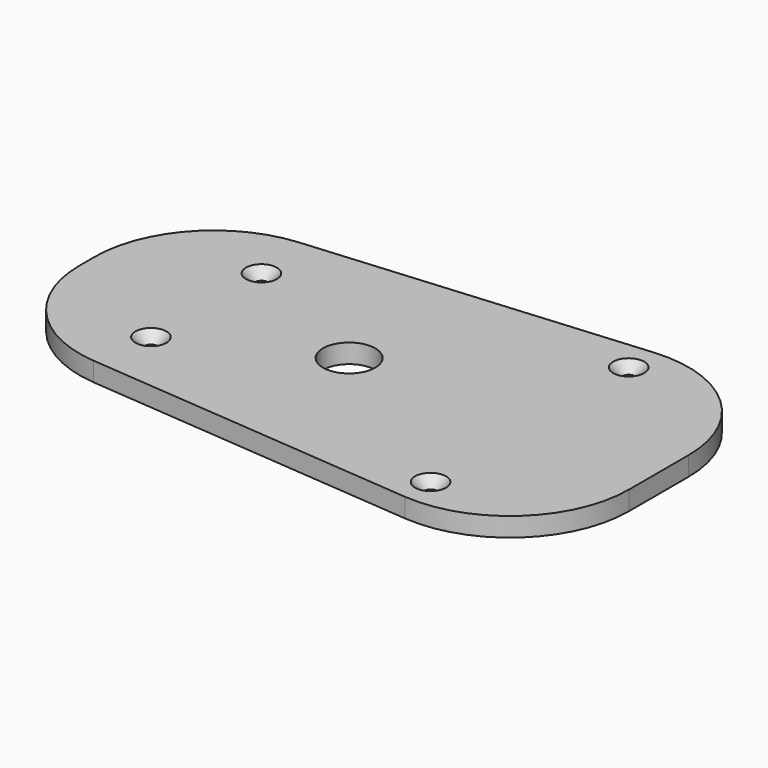
from build123d import *

# Parameters (mm, degrees)
F0_R     = 1.25
F0_R_2   = 5.5
F1_DEPTH = 4
F3_DEPTH = 2
F4_SIZE  = 2


# Not quite as in the source:
# - a feature names something its author has since deleted; it is built from what else it names


with BuildPart() as f1:
    # F0 (on Top) → F1 (new body)
    with BuildSketch(Plane.XY):
        with BuildLine():
            ThreePointArc((-36.0336562554, 5.4360876058), (-41.0336562554, 10.4360876058), (-46.0336562554, 5.4360876058))
            ThreePointArc((-46.0336562554, 5.4360876058), (-48.7113140605, 0.9910484741), (-53.6336562554, -0.6517453414))
            Line((-53.6336562554, -0.6517453414), (-57.6336562554, -0.6517453414))
            Line((-57.6336562554, -0.6517453414), (-59.4336562554, -0.6517453414))
            Line((-59.4336562554, -0.6517453414), (-59.4336562554, -1.3484233022))
            ThreePointArc((-59.4336562554, -1.3484233022), (-52.8307134237, -18.2761605269), (-36.5097932518, -26.2620672584))
            Line((-36.5097932518, -26.2620672584), (33.4902067482, -32.0954005917))
            ThreePointArc((33.4902067482, -32.0954005917), (52.4940809692, -25.5788138039), (60.5663437446, -7.1817566356))
            Line((60.5663437446, -7.1817566356), (60.5663437446, 8.4782659528))
            ThreePointArc((60.5663437446, 8.4782659528), (52.4940809692, 26.8753231211), (33.4902067482, 33.3919099089))
            Line((33.4902067482, 33.3919099089), (-36.5097932518, 27.5585765756))
            ThreePointArc((-36.5097932518, 27.5585765756), (-52.8307134237, 19.5726698441), (-59.4336562554, 2.6449326195))
            Line((-59.4336562554, 2.6449326195), (-59.4336562554, 1.9482546586))
            Line((-59.4336562554, 1.9482546586), (-57.6336562554, 1.9482546586))
            Line((-57.6336562554, 1.9482546586), (-53.6336562554, 1.9482546586))
            ThreePointArc((-53.6336562554, 1.9482546586), (-50.3543429782, 2.8450290737), (-48.4065189788, 5.6314392355))
            ThreePointArc((-48.4065189788, 5.6314392355), (-40.8279863477, 12.5929298404), (-33.4336562554, 5.4360876058))
            ThreePointArc((-33.4336562554, 5.4360876058), (-31.5267024615, 2.8420068396), (-28.4336562554, 1.9482546586))
            Line((-28.4336562554, 1.9482546586), (-15.4336562554, 1.9482546586))
            Line((-15.4336562554, 1.9482546586), (-15.4336562554, 15.2482546586))
            Line((-15.4336562554, 15.2482546586), (-4.9336562554, 15.2482546586))
            Line((-4.9336562554, 15.2482546586), (-4.9336562554, 17.1757546586))
            ThreePointArc((-4.9336562554, 17.1757546586), (-0.8336562554, 21.2757546586), (3.2663437446, 17.1757546586))
            Line((3.2663437446, 17.1757546586), (3.2663437446, 15.2482546586))
            Line((3.2663437446, 15.2482546586), (29.2163437446, 15.2482546586))
            Line((29.2163437446, 15.2482546586), (29.2163437446, 17.1757546586))
            ThreePointArc((29.2163437446, 17.1757546586), (33.3163437446, 21.2757546586), (37.4163437446, 17.1757546586))
            Line((37.4163437446, 17.1757546586), (37.4163437446, 15.2482546586))
            Line((37.4163437446, 15.2482546586), (47.9163437446, 15.2482546586))
            Line((47.9163437446, 15.2482546586), (47.9163437446, -13.9517453414))
            Line((47.9163437446, -13.9517453414), (37.4163437446, -13.9517453414))
            Line((37.4163437446, -13.9517453414), (37.4163437446, -15.8792453414))
            ThreePointArc((37.4163437446, -15.8792453414), (33.3163437446, -19.9792453414), (29.2163437446, -15.8792453414))
            Line((29.2163437446, -15.8792453414), (29.2163437446, -13.9517453414))
            Line((29.2163437446, -13.9517453414), (3.2663437446, -13.9517453414))
            Line((3.2663437446, -13.9517453414), (3.2663437446, -15.8792453414))
            ThreePointArc((3.2663437446, -15.8792453414), (-0.8336562554, -19.9792453414), (-4.9336562554, -15.8792453414))
            Line((-4.9336562554, -15.8792453414), (-4.9336562554, -13.9517453414))
            Line((-4.9336562554, -13.9517453414), (-15.4336562554, -13.9517453414))
            Line((-15.4336562554, -13.9517453414), (-15.4336562554, -0.6517453414))
            Line((-15.4336562554, -0.6517453414), (-28.4336562554, -0.6517453414))
            ThreePointArc((-28.4336562554, -0.6517453414), (-33.3559984503, 0.991048474), (-36.0336562554, 5.4360876058))
        make_face()
        with Locations((-34.4336562554, -13.8484233022)):
            Circle(F0_R, mode=Mode.SUBTRACT)
        with Locations((33.4902067482, -25.3792453414)):
            Circle(F0_R, mode=Mode.SUBTRACT)
        with Locations((-34.4336562554, 15.1449326195)):
            Circle(F0_R, mode=Mode.SUBTRACT)
        with Locations((33.4321971192, 26.6757546586)):
            Circle(F0_R, mode=Mode.SUBTRACT)
        with BuildLine():
            ThreePointArc((-53.6336562554, -0.6517453414), (-48.7113140605, 0.9910484741), (-46.0336562554, 5.4360876058))
            ThreePointArc((-46.0336562554, 5.4360876058), (-41.0336562554, 10.4360876058), (-36.0336562554, 5.4360876058))
            ThreePointArc((-36.0336562554, 5.4360876058), (-33.3559984503, 0.991048474), (-28.4336562554, -0.6517453414))
            Line((-28.4336562554, -0.6517453414), (-15.4336562554, -0.6517453414))
            Line((-15.4336562554, -0.6517453414), (-15.4336562554, -13.9517453414))
            Line((-15.4336562554, -13.9517453414), (-4.9336562554, -13.9517453414))
            Line((-4.9336562554, -13.9517453414), (-4.9336562554, -15.8792453414))
            ThreePointArc((-4.9336562554, -15.8792453414), (-0.8336562554, -19.9792453414), (3.2663437446, -15.8792453414))
            Line((3.2663437446, -15.8792453414), (3.2663437446, -13.9517453414))
            Line((3.2663437446, -13.9517453414), (29.2163437446, -13.9517453414))
            Line((29.2163437446, -13.9517453414), (29.2163437446, -15.8792453414))
            ThreePointArc((29.2163437446, -15.8792453414), (33.3163437446, -19.9792453414), (37.4163437446, -15.8792453414))
            Line((37.4163437446, -15.8792453414), (37.4163437446, -13.9517453414))
            Line((37.4163437446, -13.9517453414), (47.9163437446, -13.9517453414))
            Line((47.9163437446, -13.9517453414), (47.9163437446, 15.2482546586))
            Line((47.9163437446, 15.2482546586), (37.4163437446, 15.2482546586))
            Line((37.4163437446, 15.2482546586), (37.4163437446, 17.1757546586))
            ThreePointArc((37.4163437446, 17.1757546586), (33.3163437446, 21.2757546586), (29.2163437446, 17.1757546586))
            Line((29.2163437446, 17.1757546586), (29.2163437446, 15.2482546586))
            Line((29.2163437446, 15.2482546586), (3.2663437446, 15.2482546586))
            Line((3.2663437446, 15.2482546586), (3.2663437446, 17.1757546586))
            ThreePointArc((3.2663437446, 17.1757546586), (-0.8336562554, 21.2757546586), (-4.9336562554, 17.1757546586))
            Line((-4.9336562554, 17.1757546586), (-4.9336562554, 15.2482546586))
            Line((-4.9336562554, 15.2482546586), (-15.4336562554, 15.2482546586))
            Line((-15.4336562554, 15.2482546586), (-15.4336562554, 1.9482546586))
            Line((-15.4336562554, 1.9482546586), (-28.4336562554, 1.9482546586))
            ThreePointArc((-28.4336562554, 1.9482546586), (-31.5267024615, 2.8420068396), (-33.4336562554, 5.4360876058))
            ThreePointArc((-33.4336562554, 5.4360876058), (-40.8279863477, 12.5929298404), (-48.4065189788, 5.6314392355))
            ThreePointArc((-48.4065189788, 5.6314392355), (-50.3543429782, 2.8450290737), (-53.6336562554, 1.9482546586))
            Line((-53.6336562554, 1.9482546586), (-53.6336562554, -0.6517453414))
        make_face()
        with Locations((-4.4336562554, 0.6572546586)):
            Circle(F0_R_2, mode=Mode.SUBTRACT)
        Polygon((-59.4336562554, -0.6517453414), (-57.6336562554, -0.6517453414), (-57.6336562554, 0.6482546586), (-57.6336562554, 1.9482546586), (-59.4336562554, 1.9482546586), align=None)
        Polygon((-57.6336562554, -0.6517453414), (-53.6336562554, -0.6517453414), (-53.6336562554, 1.9482546586), (-57.6336562554, 1.9482546586), (-57.6336562554, 0.6482546586), align=None)
    extrude(amount=F1_DEPTH)

    # F2 (on face) → F3 (join)
    with BuildSketch(Plane(origin=(0, 0, 0), x_dir=(1, 0, 0), z_dir=(0, 0, -1))):
        with BuildLine():
            ThreePointArc((-53.8336562554, -1.7482546586), (-53.6922348992, -1.6896760149), (-53.6336562554, -1.5482546586))
            Line((-53.6336562554, -1.5482546586), (-53.6336562554, 0.2517453414))
            ThreePointArc((-53.6336562554, 0.2517453414), (-53.6922348992, 0.3931666976), (-53.8336562554, 0.4517453414))
            Line((-53.8336562554, 0.4517453414), (-57.4336562554, 0.4517453414))
            ThreePointArc((-57.4336562554, 0.4517453414), (-57.5750776116, 0.3931666976), (-57.6336562554, 0.2517453414))
            Line((-57.6336562554, 0.2517453414), (-57.6336562554, -0.6482546586))
            Line((-57.6336562554, -0.6482546586), (-57.6336562554, -1.5482546586))
            ThreePointArc((-57.6336562554, -1.5482546586), (-57.5750776116, -1.6896760149), (-57.4336562554, -1.7482546586))
            Line((-57.4336562554, -1.7482546586), (-53.8336562554, -1.7482546586))
        make_face()
    extrude(amount=F3_DEPTH)

    # F4
    f4_edges = [f1.edges().sort_by_distance(p)[0] for p in [
        (-35.683656, 15.144933, 4),
        (-35.683656, -13.848423, 4),
        (32.182197, 26.675755, 4),
        (32.240207, -25.379245, 4),
    ]]
    chamfer(f4_edges, length=F4_SIZE)


solid = f1.part
